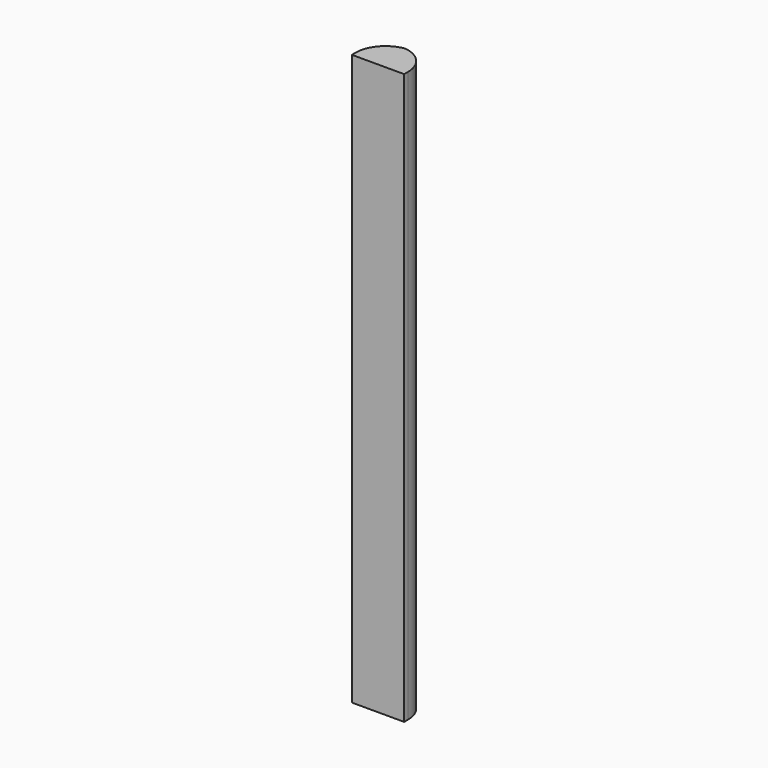
from build123d import *

# Parameters (mm, degrees)
F0_W        = 8.8490359485
F0_H        = 96.4175835252
F1_DEPTH    = 5.842
F2_T1_DEPTH = 121.8175835252


# Not quite as in the source:
# - a fillet or chamfer that OpenCascade refuses, or shapes differently, is made with other operations: its cross-section is extruded or revolved along the edge and cut away or added


with BuildPart() as f1:
    # F0 (on Front) → F1 (new body)
    with BuildSketch(Plane.XZ):
        with Locations((-62.4962914735, -2.8574988246)):
            Rectangle(F0_W, F0_H)
    extrude(amount=F1_DEPTH)

    # F2: fillet of radius 5.08 on 2 edges, made by hand

    # F2_s2 → F2_t1 (cut)
    with BuildSketch(Plane.XY.offset(-63.7662905872)):
        with BuildLine():
            ThreePointArc((-58.0717734993, -5.08), (-59.5596710508, -1.4878975516), (-63.1517734993, 0))
            Line((-63.1517734993, 0), (-58.0717734993, 0))
            Line((-58.0717734993, 0), (-58.0717734993, -5.08))
        make_face()
        with BuildLine():
            ThreePointArc((-66.9208094478, -5.08), (-65.4329118962, -1.4878975516), (-61.8408094478, 0))
            Line((-61.8408094478, 0), (-66.9208094478, 0))
            Line((-66.9208094478, 0), (-66.9208094478, -5.08))
        make_face()
    extrude(amount=F2_T1_DEPTH, mode=Mode.SUBTRACT)


solid = f1.part
